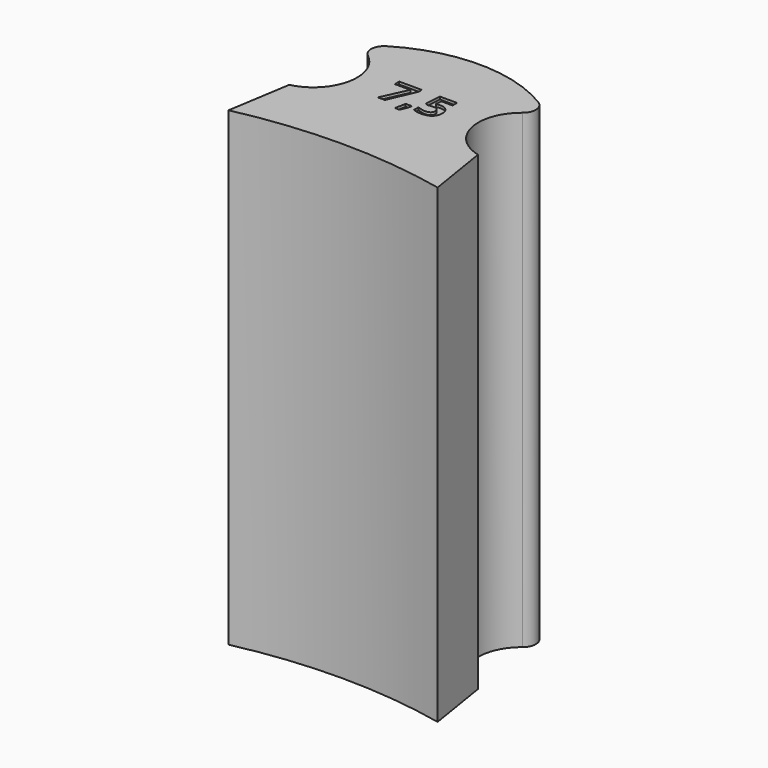
from build123d import *

# Parameters (mm, degrees)
F1_DEPTH     = 180
F2_TEXT_SIZE = 16.856395329
F3_DEPTH     = 1


# Not quite as in the source:
# - Text() gives the source's letters only with a copy of the font that has no kerning and outlines rounded to 1/6400 em; it was checked with that copy


with BuildPart() as f1:
    # F0 (on Top) → F1 (new body)
    with BuildSketch(Plane.XY):
        with BuildLine():
            Line((3.8687128108, 24.1569802165), (0, 0))
            ThreePointArc((0, 0), (40, 4.2812949374), (80, 0))
            Line((80, 0), (76.1312871892, 24.1569802165))
            ThreePointArc((76.1312871892, 24.1569802165), (63.5975554576, 36.8458138953), (69.5972800683, 53.6417728094))
            ThreePointArc((69.5972800683, 53.6417728094), (71.4969098635, 57.8715436357), (69.1043731597, 61.843359684))
            ThreePointArc((69.1043731597, 61.843359684), (40, 70), (10.8956268403, 61.843359684))
            ThreePointArc((10.8956268403, 61.843359684), (8.5030901365, 57.8715436357), (10.4027199317, 53.6417728094))
            ThreePointArc((10.4027199317, 53.6417728094), (16.4024445424, 36.8458138953), (3.8687128108, 24.1569802165))
        make_face()
    extrude(amount=F1_DEPTH)

    # F2 (on face) → F3 (cut)
    with BuildSketch(Plane.XY.offset(180)):
        with Locations((27.7659443276, 34.3472510576)):
            Text('7,5', F2_TEXT_SIZE, font='Open Sans', font_style=FontStyle.BOLD, text_align=(TextAlign.LEFT, TextAlign.BOTTOM))
    extrude(amount=-F3_DEPTH, mode=Mode.SUBTRACT)


solid = f1.part
